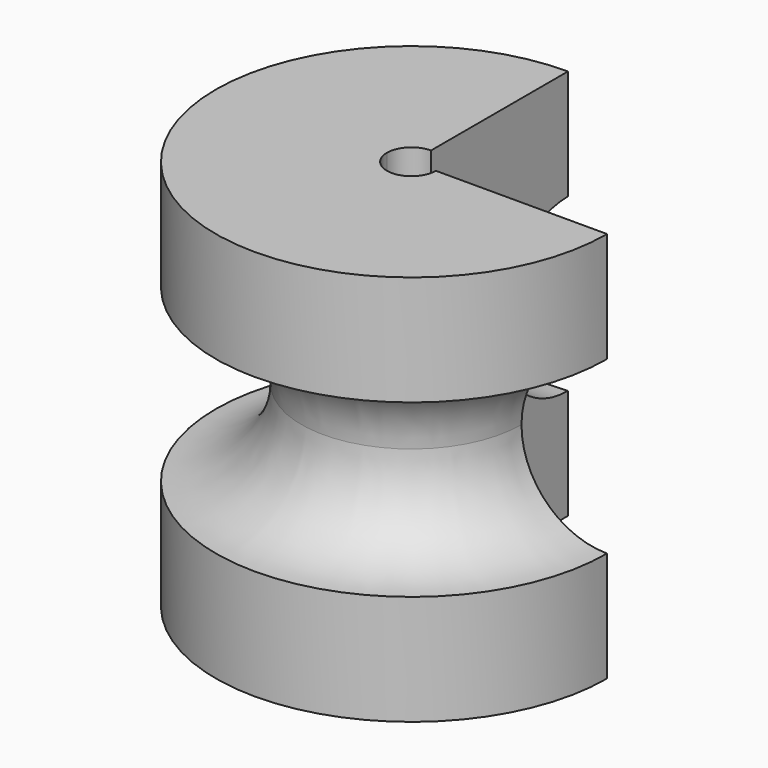
from build123d import *

# Parameters (mm, degrees)
F3_DEPTH = 25.401


with BuildPart() as f1:
    # F0 (on Front) → F1 (revolve)
    with BuildSketch(Plane.XZ):
        with BuildLine():
            Line((0, 7.14375), (0, 0))
            Line((0, 0), (12.7, 0))
            Line((12.7, 0), (12.7, 25.4))
            Line((12.7, 25.4), (0, 25.4))
            Line((0, 25.4), (0, 18.25625))
            ThreePointArc((0, 18.25625), (3.928862053, 16.628862053), (5.55625, 12.7))
            ThreePointArc((5.55625, 12.7), (3.928862053, 8.771137947), (0, 7.14375))
        make_face()
    revolve(axis=Axis((12.7, 0, 12.7), (0, 0, 1)))

    # F2 (on face) → F3 (cut, through all)
    with BuildSketch(Plane.XY.offset(25.4)):
        with BuildLine():
            Line((12.7, 1.5875), (12.7, 0))
            Line((12.7, 0), (14.2875, 0))
            ThreePointArc((14.2875, 0), (13.8225320151, 1.1225320151), (12.7, 1.5875))
        make_face()
        with BuildLine():
            Line((14.2875, 0), (12.7, 0))
            Line((12.7, 0), (11.1125, 0))
            ThreePointArc((11.1125, 0), (12.7, -1.5875), (14.2875, 0))
        make_face()
        with BuildLine():
            Line((11.1125, 0), (12.7, 0))
            Line((12.7, 0), (12.7, 1.5875))
            ThreePointArc((12.7, 1.5875), (11.5774679849, 1.1225320151), (11.1125, 0))
        make_face()
        with BuildLine():
            ThreePointArc((12.7, 1.5875), (13.8225320151, 1.1225320151), (14.2875, 0))
            Line((14.2875, 0), (25.4, 0))
            ThreePointArc((25.4, 0), (21.6802561211, 8.9802561211), (12.7, 12.7))
            Line((12.7, 12.7), (12.7, 1.5875))
        make_face()
    extrude(amount=-F3_DEPTH, mode=Mode.SUBTRACT)


solid = f1.part
